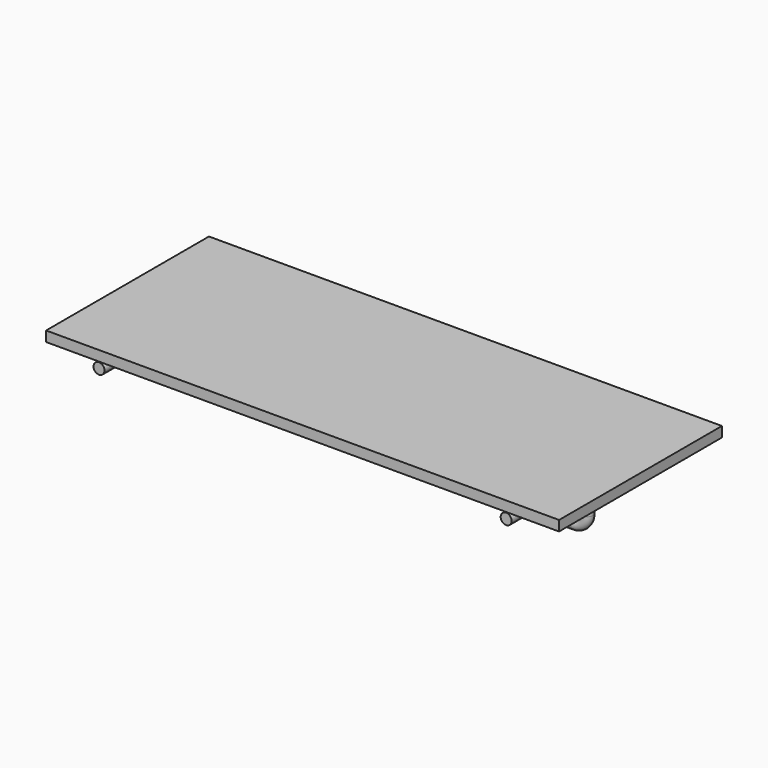
from build123d import *

# Parameters (mm, degrees)
F7_R      = 13.45
F10_R     = 13.45
F12_DEPTH = 500
F13_W     = 1260
F13_H     = 500
F14_DEPTH = 60
F15_DEPTH = 35


with BuildPart() as f8:
    # F8: sweep along a path in F4
    with BuildLine(Plane.XZ.offset(250)) as f8_path:
        Line((0, 1600), (-470, 1600))
        ThreePointArc((-470, 1600), (-491.2132034356, 1608.7867965644), (-500, 1630))
        Line((-500, 1630), (-500, 1720))
    # F7 (on Right) → F8 (sweep)
    with BuildSketch(Plane.YZ):
        with Locations((-250, 1600)):
            Circle(F7_R)
    sweep(path=f8_path.line)

    # F9: sweep along a path in F4
    with BuildLine(Plane.XZ.offset(250)) as f9_path:
        Line((0, 1600), (470, 1600))
        ThreePointArc((470, 1600), (491.2132034356, 1608.7867965644), (500, 1630))
        Line((500, 1630), (500, 1720))
    # F7 (on Right) → F9 (sweep)
    with BuildSketch(Plane.YZ):
        with Locations((-250, 1600)):
            Circle(F7_R)
    sweep(path=f9_path.line)

    # F10 (on face) → F11 (join, up to the next surface of F8)
    with BuildSketch(Plane.XZ):
        with Locations((0, 1600)):
            Circle(F10_R)
    extrude(until=Until.NEXT)

    # F10 (on face) → F12 (join)
    with BuildSketch(Plane.XZ):
        with Locations((-500, 1720)):
            Circle(F10_R)
        with Locations((500, 1720)):
            Circle(F10_R)
    extrude(amount=F12_DEPTH)


with BuildPart() as f14:
    # F13 (on offset) → F14 (new body)
    with BuildSketch(Plane.XY.offset(1700)):
        with Locations((0, -250)):
            Rectangle(F13_W, F13_H)
    extrude(amount=F14_DEPTH)

    # F13 (on offset) → F15 (cut)
    with BuildSketch(Plane.XY.offset(1700)):
        with Locations((0, -250)):
            Rectangle(F13_W, F13_H)
    extrude(amount=F15_DEPTH, mode=Mode.SUBTRACT)


solid = Compound([f8.part, f14.part])
